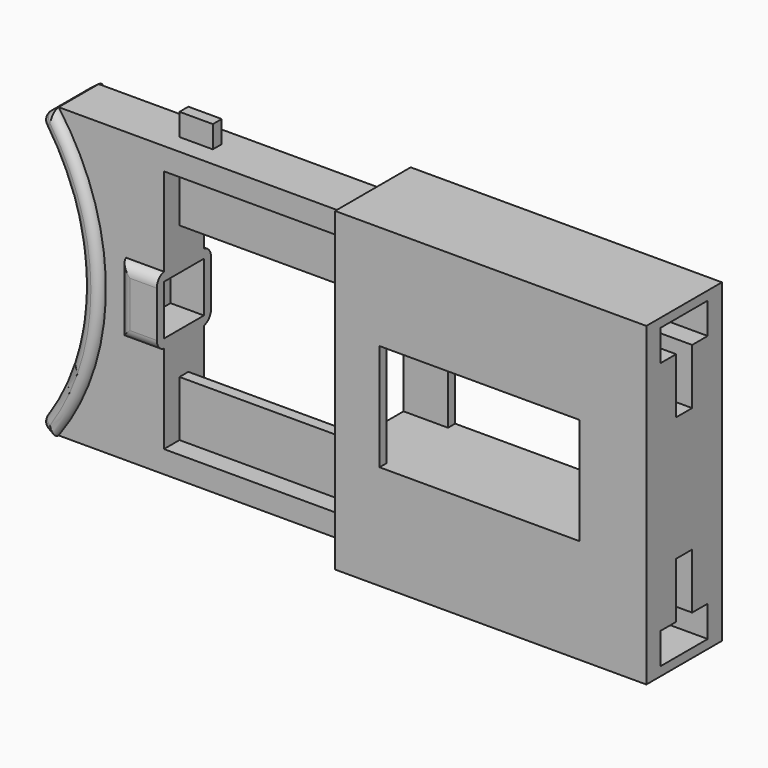
from build123d import *

# Parameters (mm, degrees)
F1_DEPTH    = 2.25
F2_W        = 6.1
F2_H        = 6.1
F2_W_2      = 4.5
F2_H_2      = 4.5
F3_DEPTH    = 3.4
F5_DEPTH    = 3
F6_R        = 0.74999
F7_T1_DEPTH = 10.9989794856
F7_T3_DEPTH = 5.8494897428
F9_DEPTH    = 17
F10_W       = 3
F10_H       = 1
F11_DEPTH   = 2
F12_W       = 8.5
F12_H       = 28.4
F12_W_2     = 6.9
F12_H_2     = 9.6
F13_DEPTH   = 28
F15_W       = 22
F15_H       = 9.6
F16_DEPTH   = 15.5
F17_DEPTH   = 6
F19_DEPTH   = 5


# Not quite as in the source:
# - a fillet or chamfer that OpenCascade refuses, or shapes differently, is made with other operations: its cross-section is extruded or revolved along the edge and cut away or added
# - a fillet or chamfer is up to 0.001 mm smaller than in the source, because OpenCascade refuses the exact size


with BuildPart() as f1:
    # F0 (on Front) → F1 (new body, symmetric)
    with BuildSketch(Plane.XZ):
        with BuildLine():
            Line((-9.5380139407, -2.7482741908), (-9.5380139407, 1.7517258092))
            Line((-9.5380139407, 1.7517258092), (-6.5380139407, 1.7517258092))
            Line((-6.5380139407, 1.7517258092), (-6.5380139407, 4.7517258092))
            Line((-6.5380139407, 4.7517258092), (10.4619860593, 4.7517258092))
            Line((10.4619860593, 4.7517258092), (10.4619860593, 12.5017258092))
            Line((10.4619860593, 12.5017258092), (-16.0051570773, 12.5017258092))
            ThreePointArc((-16.0051570773, 12.5017258092), (-11.7548404249, -0.4982741908), (-16.0051570773, -13.4982741908))
            Line((-16.0051570773, -13.4982741908), (10.4619860593, -13.4982741908))
            Line((10.4619860593, -13.4982741908), (10.4619860593, -5.7482741908))
            Line((10.4619860593, -5.7482741908), (-6.5380139407, -5.7482741908))
            Line((-6.5380139407, -5.7482741908), (-6.5380139407, -2.7482741908))
            Line((-6.5380139407, -2.7482741908), (-9.5380139407, -2.7482741908))
        make_face()
    extrude(amount=F1_DEPTH, both=True)

    # F2 (on face) → F3 (join)
    with BuildSketch(Plane.YZ.offset(-6.5380139407)):
        with Locations((0, -0.4982741908)):
            Rectangle(F2_W, F2_H)
        with Locations((0, -0.4982741908)):
            Rectangle(F2_W_2, F2_H_2, mode=Mode.SUBTRACT)
    extrude(amount=-F3_DEPTH)

    # F4 (on Front) → F5 (join, symmetric)
    with BuildSketch(Plane.XZ):
        with BuildLine():
            ThreePointArc((-16.0051570773, -13.4982741908), (-11.7548404249, -0.4982741908), (-16.0051570773, 12.5017258092))
            Line((-16.0051570773, 12.5017258092), (-17.2154421685, 11.6156050511))
            ThreePointArc((-17.2154421685, 11.6156050511), (-13.2548404249, -0.4982741908), (-17.2154421685, -12.6121534326))
            Line((-17.2154421685, -12.6121534326), (-16.0051570773, -13.4982741908))
        make_face()
    extrude(amount=F5_DEPTH, both=True)

    # F6 (radius 0.75 in the source; OpenCascade refuses exactly that, so slightly less here)
    f6_edges = [f1.edges().sort_by_distance(p)[0] for p in [
        (-16.6103, -3, 12.058665),
        (-13.25484, -3, -0.498274),
        (-16.6103, -3, -13.055214),
        (-11.75484, -3, -0.498274),
        (-16.6103, 3, 12.058665),
        (-13.25484, 3, -0.498274),
        (-16.6103, 3, -13.055214),
        (-11.75484, 3, -0.498274),
        (-17.215442, 0, -12.612153),
        (-17.215442, 0, 11.615605),
    ]]
    fillet(f6_edges, radius=F6_R)

    # F7: fillet of radius 1 on 6 edges, made by hand

    # F7_s2 → F7_t1 (cut)
    with BuildSketch(Plane.XY.offset(-5.9977639336)):
        with BuildLine():
            ThreePointArc((-9.9380139407, -2.25), (-9.5906735756, -2.8245966692), (-8.9582180436, -3.05))
            Line((-8.9582180436, -3.05), (-9.9380139407, -3.05))
            Line((-9.9380139407, -3.05), (-9.9380139407, -2.25))
        make_face()
        with BuildLine():
            ThreePointArc((-9.9380139407, 2.25), (-9.5906735756, 2.8245966692), (-8.9582180436, 3.05))
            Line((-8.9582180436, 3.05), (-9.9380139407, 3.05))
            Line((-9.9380139407, 3.05), (-9.9380139407, 2.25))
        make_face()
    extrude(amount=F7_T1_DEPTH, mode=Mode.SUBTRACT)

    # F7_s4 → F7_t3 (cut)
    with BuildSketch(Plane.YZ.offset(-9.9380139407)):
        with BuildLine():
            ThreePointArc((-2.25, -3.5482741908), (-2.8245966692, -3.2009338257), (-3.05, -2.5684782937))
            Line((-3.05, -2.5684782937), (-3.05, -3.5482741908))
            Line((-3.05, -3.5482741908), (-2.25, -3.5482741908))
        make_face()
        with BuildLine():
            ThreePointArc((-2.25, 2.5517258092), (-2.8245966692, 2.2043854441), (-3.05, 1.5719299121))
            Line((-3.05, 1.5719299121), (-3.05, 2.5517258092))
            Line((-3.05, 2.5517258092), (-2.25, 2.5517258092))
        make_face()
        with BuildLine():
            ThreePointArc((2.25, 2.5517258092), (2.8245966692, 2.2043854441), (3.05, 1.5719299121))
            Line((3.05, 1.5719299121), (3.05, 2.5517258092))
            Line((3.05, 2.5517258092), (2.25, 2.5517258092))
        make_face()
        with BuildLine():
            ThreePointArc((2.25, -3.5482741908), (2.8245966692, -3.2009338257), (3.05, -2.5684782937))
            Line((3.05, -2.5684782937), (3.05, -3.5482741908))
            Line((3.05, -3.5482741908), (2.25, -3.5482741908))
        make_face()
    extrude(amount=F7_T3_DEPTH, mode=Mode.SUBTRACT)

    # F8 (on face) → F9 (cut, through all)
    with BuildSketch(Plane.YZ.offset(10.4619860593)):
        Polygon((-2.25, 10.5017258092), (-2.25, 4.7517258092), (2.25, 4.7517258092), (2.25, 10.5017258092), (0.5, 10.5017258092), (0.5, 5.5017258092), (-0.5, 5.5017258092), (-0.5, 10.5017258092), align=None)
        Polygon((2.25, -11.4982741908), (2.25, -5.7482741908), (-2.25, -5.7482741908), (-2.25, -11.4982741908), (-0.5, -11.4982741908), (-0.5, -6.4982741908), (0.5, -6.4982741908), (0.5, -11.4982741908), align=None)
    extrude(amount=-F9_DEPTH, mode=Mode.SUBTRACT)

    # F10 (on face) → F11 (join)
    with BuildSketch(Plane.XY.offset(12.5017258092)):
        with Locations((-5.0380139407, 0)):
            Rectangle(F10_W, F10_H)
    extrude(amount=F11_DEPTH)


with BuildPart() as f13:
    # F12 (on face) → F13 (new body)
    with BuildSketch(Plane.YZ.offset(10.4619860593)):
        with Locations((0, -0.4982741908)):
            Rectangle(F12_W, F12_H)
        Polygon((-0.9, -6.0982741908), (0.9, -6.0982741908), (0.9, -11.0982741908), (2.65, -11.0982741908), (2.65, -13.8982741908), (-2.65, -13.8982741908), (-2.65, -11.0982741908), (-0.9, -11.0982741908), align=None, mode=Mode.SUBTRACT)
        with Locations((0, -0.4982741908)):
            Rectangle(F12_W_2, F12_H_2, mode=Mode.SUBTRACT)
        Polygon((0.9, 10.1017258092), (0.9, 5.1017258092), (-0.9, 5.1017258092), (-0.9, 10.1017258092), (-2.65, 10.1017258092), (-2.65, 12.9017258092), (2.65, 12.9017258092), (2.65, 10.1017258092), align=None, mode=Mode.SUBTRACT)
    extrude(amount=F13_DEPTH)

    # F15 (on face) → F16 (cut)
    with BuildSketch(Plane(origin=(0, 4.25, 0), x_dir=(-1, 0, 0), z_dir=(0, 1, 0))):
        with Locations((-25.4619860593, -0.4982741908)):
            Rectangle(F15_W, F15_H)
    extrude(amount=-F16_DEPTH, mode=Mode.SUBTRACT)

    # F14 (on face) → F17 (join)
    with BuildSketch(Plane.YZ.offset(38.4619860593)):
        Polygon((3.45, 4.3017258092), (-3.45, 4.3017258092), (-4.25, 4.3017258092), (-4.25, -5.2982741908), (-3.45, -5.2982741908), (3.45, -5.2982741908), (4.25, -5.2982741908), (4.25, 4.3017258092), align=None)
    extrude(amount=-F17_DEPTH)

    # F18 (on face) → F19 (cut)
    with BuildSketch(Plane(origin=(32.4619860593, 0, 0), x_dir=(0, -1, 0), z_dir=(-1, 0, 0))):
        with BuildLine():
            ThreePointArc((-3.0923292192, -1), (0.5061768651, -3.2103403217), (3.25, 0))
            ThreePointArc((3.25, 0), (0.5061768651, 3.2103403217), (-3.0923292192, 1))
            ThreePointArc((-3.0923292192, 1), (-3.25, 0), (-3.0923292192, -1))
        make_face()
        with BuildLine():
            ThreePointArc((-3.0923292192, -1), (-3.25, 0), (-3.0923292192, 1))
            Line((-3.0923292192, 1), (-4.25, 1))
            Line((-4.25, 1), (-4.25, -1))
            Line((-4.25, -1), (-3.0923292192, -1))
        make_face()
    extrude(amount=-F19_DEPTH, mode=Mode.SUBTRACT)


solid = Compound([f1.part, f13.part])
